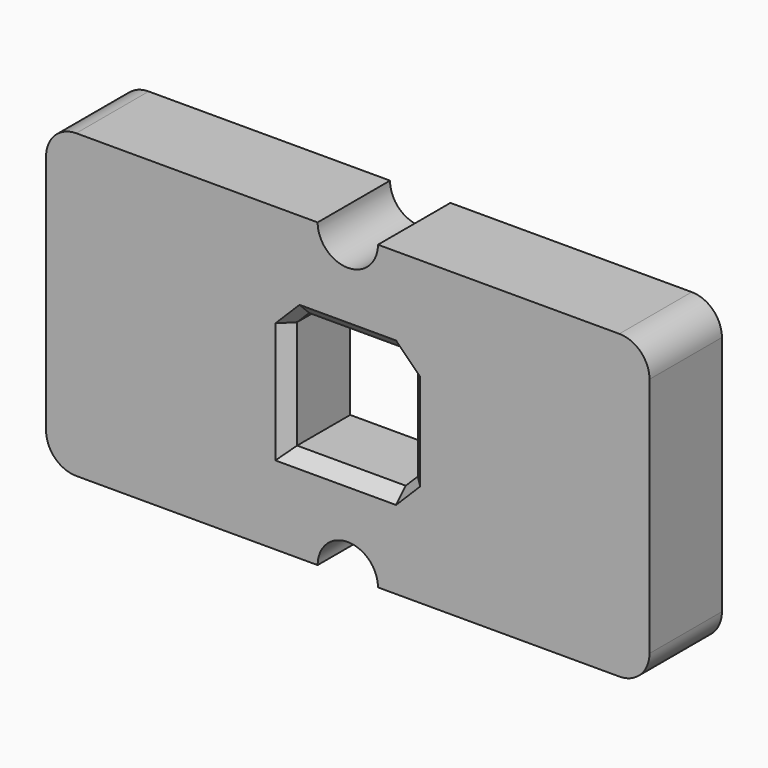
from build123d import *

# Parameters (mm, degrees)
F0_W     = 50.8
F0_H     = 50.8
F1_DEPTH = 38.1
F2_SIZE  = 5.08


with BuildPart() as f1:
    # F0 (on Front) → F1 (new body)
    with BuildSketch(Plane.XZ):
        with BuildLine():
            Line((-14.8284427494, 76.4413994114), (-116.4284427494, 76.4413994114))
            ThreePointArc((-116.4284427494, 76.4413994114), (-125.4086988705, 72.7216555324), (-129.1284427494, 63.7413994114))
            Line((-129.1284427494, 63.7413994114), (-129.1284427494, -37.8586005886))
            ThreePointArc((-129.1284427494, -37.8586005886), (-125.4086988705, -46.8388567097), (-116.4284427494, -50.5586005886))
            Line((-116.4284427494, -50.5586005886), (-14.8284427494, -50.5586005886))
            ThreePointArc((-14.8284427494, -50.5586005886), (-2.1284427494, -37.8586005886), (10.5715572506, -50.5586005886))
            Line((10.5715572506, -50.5586005886), (112.1715572506, -50.5586005886))
            ThreePointArc((112.1715572506, -50.5586005886), (121.1518133717, -46.8388567097), (124.8715572506, -37.8586005886))
            Line((124.8715572506, -37.8586005886), (124.8715572506, 63.7413994114))
            ThreePointArc((124.8715572506, 63.7413994114), (121.1518133717, 72.7216555324), (112.1715572506, 76.4413994114))
            Line((112.1715572506, 76.4413994114), (10.5715572506, 76.4413994114))
            ThreePointArc((10.5715572506, 76.4413994114), (-2.1284427494, 63.7413994114), (-14.8284427494, 76.4413994114))
        make_face()
        with Locations((-2.1284427494, 12.9413994114)):
            Rectangle(F0_W, F0_H, mode=Mode.SUBTRACT)
    extrude(amount=F1_DEPTH)

    # F2
    f2_edges = [f1.edges().sort_by_distance(p)[0] for p in [
        (23.271557, -19.05, 38.341399),
        (23.271557, -19.05, -12.458601),
        (23.271557, 0, 12.941399),
        (23.271557, -38.1, 12.941399),
        (-27.528443, -19.05, 38.341399),
        (-2.128443, 0, 38.341399),
        (-2.128443, -38.1, 38.341399),
        (-27.528443, 0, 12.941399),
        (-27.528443, -38.1, 12.941399),
        (-2.128443, 0, -12.458601),
        (-2.128443, -38.1, -12.458601),
    ]]
    chamfer(f2_edges, length=F2_SIZE)


solid = f1.part
